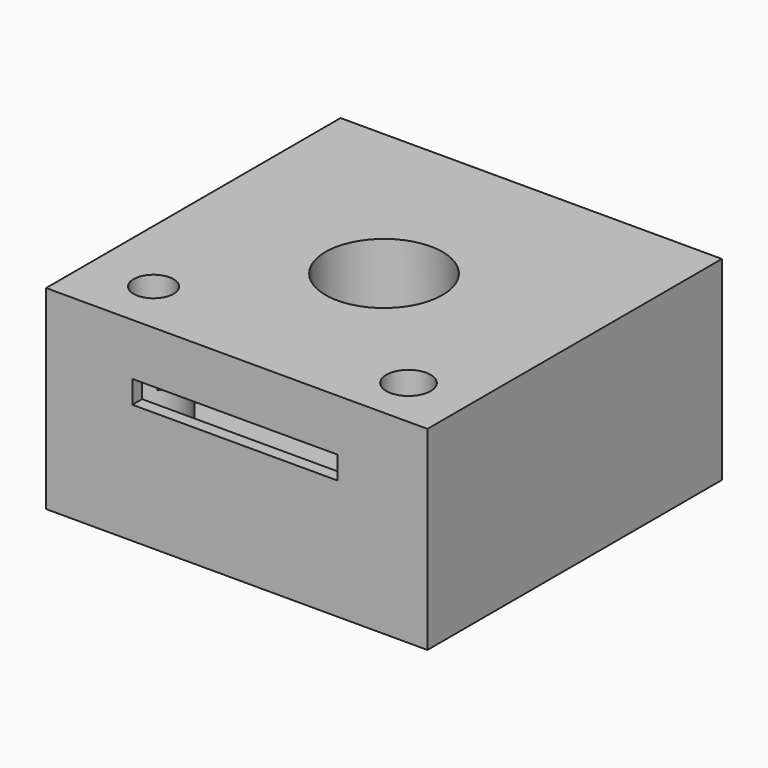
from build123d import *

# Parameters (mm, degrees)
F0_W         = 78.3775448799
F0_H         = 75.6465569139
F1_DEPTH     = 25
F2_R         = 12.0203528279
F3_DEPTH     = 49.9
F4_T         = -2.5
F5_R         = 6.6018014855
F6_DEPTH     = 25
F7_T         = 2.5
F7_T3_DEPTH  = 27.5
F7_T5_DEPTH  = 78.3775448799
F7_T7_DEPTH  = 75.6465569139
F8_DEPTH     = 25
F9_R         = 7.0468826158
F10_DEPTH    = 25
F11_T        = 2.5
F11_T3_DEPTH = 27.5
F11_T5_DEPTH = 78.3775448799
F11_T7_DEPTH = 75.6465569139
F12_DEPTH    = 25
F13_W        = 42.1091411263
F13_H        = 4.6861004084
F14_DEPTH    = 25
F15_W        = 78.3775448799
F15_H        = 75.6465569139
F16_DEPTH    = 15
F17_R        = 10.5957056812
F18_DEPTH    = 25
F19_DEPTH    = 25
F20_DEPTH    = 25
F21_DEPTH    = 25


# Not quite as in the source:
# - a shell that OpenCascade refuses in one call is made with other operations: the cavity is built on its own and cut out


with BuildPart() as f1:
    # F0 (on Top) → F1 (new body)
    with BuildSketch(Plane.XY):
        Rectangle(F0_W, F0_H)
    extrude(amount=F1_DEPTH)

    # F2 (on face) → F3 (cut)
    with BuildSketch(Plane(origin=(0, 0, 0), x_dir=(1, 0, 0), z_dir=(0, 0, -1))):
        Circle(F2_R)
    extrude(amount=-F3_DEPTH, mode=Mode.SUBTRACT)

    # F4
    f4_openings = [f1.faces().sort_by_distance(p)[0] for p in [
        (0, 36.733992, 0),
    ]]
    offset(amount=F4_T, openings=f4_openings)

    # F5 (on face) → F6 (join)
    with BuildSketch(Plane(origin=(0, 0, 22.5), x_dir=(1, 0, 0), z_dir=(0, 0, -1))):
        with Locations((-26.0466337204, 26.645489037)):
            Circle(F5_R)
    extrude(amount=F6_DEPTH)

    # F7: shell of thickness 2.5, made by hand


with BuildPart() as f7_core1:
    # F7_t2: copy of F1
    add(f1.part)

    # the walls: a layer under each face that stays
    f7_faces = [f7_core1.faces().sort_by_distance(p)[0] for p in [
        (0, 37.8232784569, 12.5),
        (39.18877244, 0, 12.5),
        (-39.18877244, 0, 12.5),
        (-36.7394741625, 7.0043108254, 0),
        (-26.1258482933, -25.2155189713, 25),
        (0, -37.8232784569, 12.5),
        (0, 35.3232784569, 11.25),
        (36.68877244, 0, 11.25),
        (0, -35.3232784569, 11.25),
        (-36.68877244, 0, 11.25),
        (-12.0203528279, 0, 12.5),
        (-24.4591816266, 0, 22.5),
        (-9.6802352186, -9.6802352186, 0),
        (-32.6484352059, -26.645489037, 10),
        (-14.5203528279, 0, 11.25),
    ]]
    thicken(f7_faces, amount=-F7_T, mode=Mode.SUBTRACT)

    # F7_s4 → F7_t3 (cut)
    with BuildSketch(Plane.XY.offset(-2.5)):
        Polygon((36.66377244, 35.2982784569), (36.68877244, 37.8232784569), (39.18877244, 37.8232784569), (39.18877244, 35.3232784569), align=None)
        Polygon((-36.66377244, 35.2982784569), (-36.68877244, 37.8232784569), (-39.18877244, 37.8232784569), (-39.18877244, 35.3232784569), align=None)
        Polygon((36.66377244, -35.2982784569), (39.18877244, -35.3232784569), (39.18877244, -37.8232784569), (36.68877244, -37.8232784569), align=None)
        Polygon((-36.66377244, -35.2982784569), (-36.68877244, -37.8232784569), (-39.18877244, -37.8232784569), (-39.18877244, -35.3232784569), align=None)
    extrude(amount=F7_T3_DEPTH, mode=Mode.SUBTRACT)

    # F7_s6 → F7_t5 (cut)
    with BuildSketch(Plane.YZ.offset(-39.18877244)):
        Polygon((35.2982784569, 22.475), (37.8232784569, 22.5), (37.8232784569, 25), (35.3232784569, 25), align=None)
        Polygon((-35.2982784569, 22.475), (-37.8232784569, 22.5), (-37.8232784569, 25), (-35.3232784569, 25), align=None)
    extrude(amount=F7_T5_DEPTH, mode=Mode.SUBTRACT)

    # F7_s8 → F7_t7 (cut)
    with BuildSketch(Plane.XZ.offset(-37.8232784569)):
        Polygon((36.66377244, 22.475), (39.18877244, 22.5), (39.18877244, 25), (36.68877244, 25), align=None)
        Polygon((-36.66377244, 22.475), (-39.18877244, 22.5), (-39.18877244, 25), (-36.68877244, 25), align=None)
    extrude(amount=F7_T7_DEPTH, mode=Mode.SUBTRACT)

    # F7_s9 → F7_t10 (revolve, cut)
    with BuildSketch(Plane.XZ.offset(26.645489037)):
        Polygon((-19.4198322349, 22.475), (-19.4448322349, 25), (-21.9448322349, 25), (-21.9448322349, 22.5), align=None)
    revolve(axis=Axis((-26.0466337204, -26.645489037, 22.5), (0, 0, -1)), mode=Mode.SUBTRACT)

    # F7_s11 → F7_t12 (revolve, cut)
    with BuildSketch(Plane.XZ):
        Polygon((14.5453528279, 22.475), (14.5203528279, 25), (12.0203528279, 25), (12.0203528279, 22.5), align=None)
    revolve(axis=Axis((0, 0, 22.5), (0, 0, -1)), mode=Mode.SUBTRACT)


with BuildPart() as f1_1:
    add(f1.part)

    # what is left inside the walls is the cavity
    f7_cavity = [f7_core1.part.solids().sort_by_distance(p)[0] for p in [
        (-30.123435, -26.645489, 5.833333),
    ]]
    add(f7_cavity, mode=Mode.SUBTRACT)

    # F8 (cut): a face of the model
    f8_faces = [f1_1.faces().sort_by_distance(p)[0] for p in [
        (-26.0466337204, -26.645489037, 22.5),
    ]]
    extrude(f8_faces, amount=-F8_DEPTH, mode=Mode.SUBTRACT)

    # F9 (on face) → F10 (join)
    with BuildSketch(Plane(origin=(0, 0, 22.5), x_dir=(1, 0, 0), z_dir=(0, 0, -1))):
        with Locations((26.8326979131, 27.2501390427)):
            Circle(F9_R)
    extrude(amount=F10_DEPTH)

    # F11: shell of thickness 2.5, made by hand


with BuildPart() as f11_core1:
    # F11_t2: copy of F1
    add(f1_1.part)

    # the walls: a layer under each face that stays
    f11_faces = [f11_core1.faces().sort_by_distance(p)[0] for p in [
        (0, 37.8232784569, 12.5),
        (39.18877244, 0, 12.5),
        (-39.18877244, 0, 12.5),
        (-36.7394741625, 7.0043108254, 0),
        (-26.1258482933, 0, 25),
        (0, -37.8232784569, 12.5),
        (0, 35.3232784569, 11.25),
        (36.68877244, 0, 11.25),
        (0, -35.3232784569, 11.25),
        (-36.68877244, 0, 11.25),
        (-30.1484352059, -26.645489037, 23.75),
        (-12.0203528279, 0, 12.5),
        (-24.4591816266, 0, 22.5),
        (-30.1484352059, -26.645489037, 10),
        (-9.6802352186, -9.6802352186, 0),
        (-32.6484352059, -26.645489037, 10),
        (19.7858152973, -27.2501390427, 10),
        (-14.5203528279, 0, 11.25),
        (-30.4478347107, -22.2442880467, -2.5),
    ]]
    thicken(f11_faces, amount=-F11_T, mode=Mode.SUBTRACT)

    # F11_s4 → F11_t3 (cut)
    with BuildSketch(Plane.XY.offset(-2.5)):
        Polygon((36.66377244, 35.2982784569), (36.68877244, 37.8232784569), (39.18877244, 37.8232784569), (39.18877244, 35.3232784569), align=None)
        Polygon((-36.66377244, 35.2982784569), (-36.68877244, 37.8232784569), (-39.18877244, 37.8232784569), (-39.18877244, 35.3232784569), align=None)
        Polygon((36.66377244, -35.2982784569), (39.18877244, -35.3232784569), (39.18877244, -37.8232784569), (36.68877244, -37.8232784569), align=None)
        Polygon((-36.66377244, -35.2982784569), (-36.68877244, -37.8232784569), (-39.18877244, -37.8232784569), (-39.18877244, -35.3232784569), align=None)
    extrude(amount=F11_T3_DEPTH, mode=Mode.SUBTRACT)

    # F11_s6 → F11_t5 (cut)
    with BuildSketch(Plane.YZ.offset(-39.18877244)):
        Polygon((35.2982784569, 22.475), (37.8232784569, 22.5), (37.8232784569, 25), (35.3232784569, 25), align=None)
        Polygon((-35.2982784569, 22.475), (-37.8232784569, 22.5), (-37.8232784569, 25), (-35.3232784569, 25), align=None)
    extrude(amount=F11_T5_DEPTH, mode=Mode.SUBTRACT)

    # F11_s8 → F11_t7 (cut)
    with BuildSketch(Plane.XZ.offset(-37.8232784569)):
        Polygon((36.66377244, 22.475), (39.18877244, 22.5), (39.18877244, 25), (36.68877244, 25), align=None)
        Polygon((-36.66377244, 22.475), (-39.18877244, 22.5), (-39.18877244, 25), (-36.68877244, 25), align=None)
    extrude(amount=F11_T7_DEPTH, mode=Mode.SUBTRACT)

    # F11_s9 → F11_t10 (revolve, cut)
    with BuildSketch(Plane.XZ.offset(26.645489037)):
        Polygon((-19.4198322349, 22.475), (-19.4448322349, 25), (-21.9448322349, 25), (-21.9448322349, 22.5), align=None)
    revolve(axis=Axis((-26.0466337204, -26.645489037, 22.5), (0, 0, -1)), mode=Mode.SUBTRACT)

    # F11_s11 → F11_t12 (revolve, cut)
    with BuildSketch(Plane.XZ.offset(27.2501390427)):
        Polygon((33.9045805288, 22.475), (33.8795805288, 25), (31.3795805288, 25), (31.3795805288, 22.5), align=None)
    revolve(axis=Axis((26.8326979131, -27.2501390427, 22.5), (0, 0, -1)), mode=Mode.SUBTRACT)

    # F11_s13 → F11_t14 (revolve, cut)
    with BuildSketch(Plane.XZ):
        Polygon((14.5453528279, 22.475), (14.5203528279, 25), (12.0203528279, 25), (12.0203528279, 22.5), align=None)
    revolve(axis=Axis((0, 0, 22.5), (0, 0, -1)), mode=Mode.SUBTRACT)


with BuildPart() as f1_2:
    add(f1_1.part)

    # what is left inside the walls is the cavity
    f11_cavity = [f11_core1.part.solids().sort_by_distance(p)[0] for p in [
        (22.310815, -27.250139, 5.833333),
    ]]
    add(f11_cavity, mode=Mode.SUBTRACT)

    # F12 (cut): a face of the model
    f12_faces = [f1_2.faces().sort_by_distance(p)[0] for p in [
        (26.8326979131, -27.2501390427, 22.5),
    ]]
    extrude(f12_faces, amount=-F12_DEPTH, mode=Mode.SUBTRACT)

    # F13 (on face) → F14 (cut)
    with BuildSketch(Plane.XZ.offset(37.8232784569)):
        with Locations((-0.3970777616, 11.9879292324)):
            Rectangle(F13_W, F13_H)
    extrude(amount=-F14_DEPTH, mode=Mode.SUBTRACT)

    # F15 (on face) → F16 (join)
    with BuildSketch(Plane(origin=(0, 0, 0), x_dir=(1, 0, 0), z_dir=(0, 0, -1))):
        Rectangle(F15_W, F15_H)
    extrude(amount=F16_DEPTH)

    # F17 (on face) → F18 (cut)
    with BuildSketch(Plane(origin=(0, 0, -15), x_dir=(1, 0, 0), z_dir=(0, 0, -1))):
        with Locations((-27.1771177649, 22.4702265114)):
            Circle(F17_R)
    extrude(amount=F18_DEPTH, mode=Mode.SUBTRACT)

    # F19 (cut): a face of the model
    f19_faces = [f1_2.faces().sort_by_distance(p)[0] for p in [
        (0, 0, 0),
    ]]
    extrude(f19_faces, amount=-F19_DEPTH, mode=Mode.SUBTRACT)

    # F20 (cut): a face of the model
    f20_faces = [f1_2.faces().sort_by_distance(p)[0] for p in [
        (-26.0466337204, -26.645489037, 0),
    ]]
    extrude(f20_faces, amount=-F20_DEPTH, mode=Mode.SUBTRACT)

    # F21 (cut): a face of the model
    f21_faces = [f1_2.faces().sort_by_distance(p)[0] for p in [
        (26.8326979131, -27.2501390427, 0),
    ]]
    extrude(f21_faces, amount=-F21_DEPTH, mode=Mode.SUBTRACT)


solid = f1_2.part
